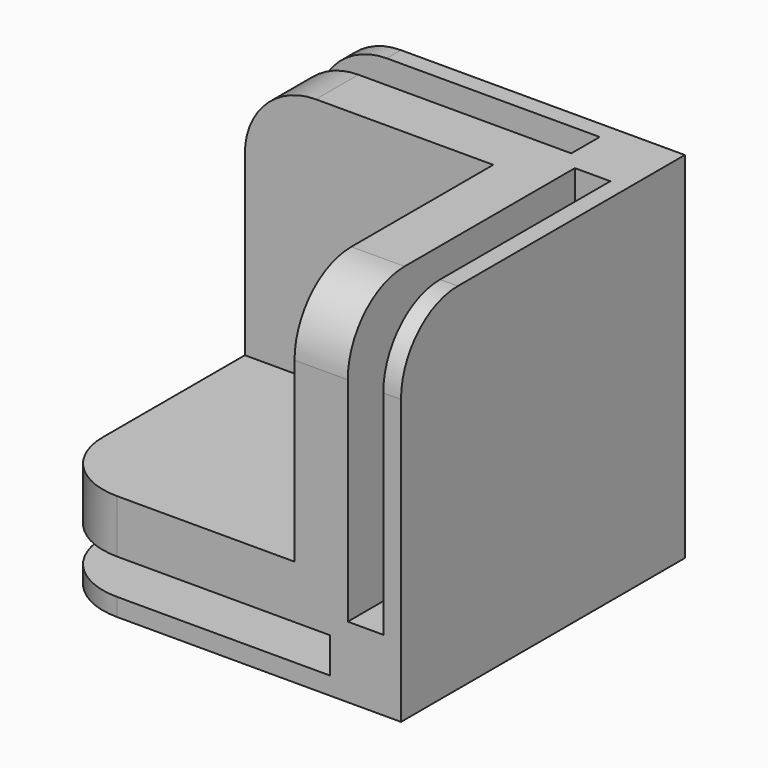
from build123d import *

# Parameters (mm, degrees)
F1_DEPTH = 15
F3_DEPTH = 15
F5_DEPTH = 15
F6_W     = 20
F6_H     = 5
F6_W_2   = 5
F6_H_2   = 30
F6_H_3   = 20
F7_DEPTH = 40
F8_W     = 30
F8_H     = 5
F8_W_2   = 20
F9_DEPTH = 40


# Not quite as in the source:
# - a feature names something its author has since deleted; it is built from what else it names


with BuildPart() as f1:
    # F0 (on Top) → F1 (new body)
    with BuildSketch(Plane.XY):
        with BuildLine():
            Line((0, -50), (0, 0))
            Line((0, 0), (-50, 0))
            Line((-50, 0), (-50, -40))
            ThreePointArc((-50, -40), (-47.0710678119, -47.0710678119), (-40, -50))
            Line((-40, -50), (0, -50))
        make_face()
    extrude(amount=F1_DEPTH)

    # F2 (on Right) → F3 (join)
    with BuildSketch(Plane.YZ):
        with BuildLine():
            Line((-50, 10), (0, 10))
            Line((0, 10), (0, 50))
            Line((0, 50), (-40, 50))
            ThreePointArc((-40, 50), (-47.0710678119, 47.0710678119), (-50, 40))
            Line((-50, 40), (-50, 10))
        make_face()
    extrude(amount=-F3_DEPTH)

    # F4 (on Front) → F5 (join)
    with BuildSketch(Plane.XZ):
        with BuildLine():
            Line((-50, 10), (-10, 10))
            Line((-10, 10), (-10, 50))
            Line((-10, 50), (-40, 50))
            ThreePointArc((-40, 50), (-47.0710678119, 47.0710678119), (-50, 40))
            Line((-50, 40), (-50, 10))
        make_face()
    extrude(amount=F5_DEPTH)

    # F6 (on face) → F7 (cut)
    with BuildSketch(Plane.XZ.offset(50)):
        Polygon((-15, 2.5), (-10, 2.5), (-10, 7.5), (-40, 7.5), (-40, 2.5), align=None)
        with Locations((-50, 5)):
            Rectangle(F6_W, F6_H)
        with Locations((-5, 25)):
            Rectangle(F6_W_2, F6_H_2)
        with Locations((-5, 50)):
            Rectangle(F6_W_2, F6_H_3)
    extrude(amount=-F7_DEPTH, mode=Mode.SUBTRACT)

    # F8 (on face) → F9 (cut)
    with BuildSketch(Plane.XY.offset(50)):
        with Locations((-25, -5)):
            Rectangle(F8_W, F8_H)
        with Locations((-50, -5)):
            Rectangle(F8_W_2, F8_H)
    extrude(amount=-F9_DEPTH, mode=Mode.SUBTRACT)


solid = f1.part
